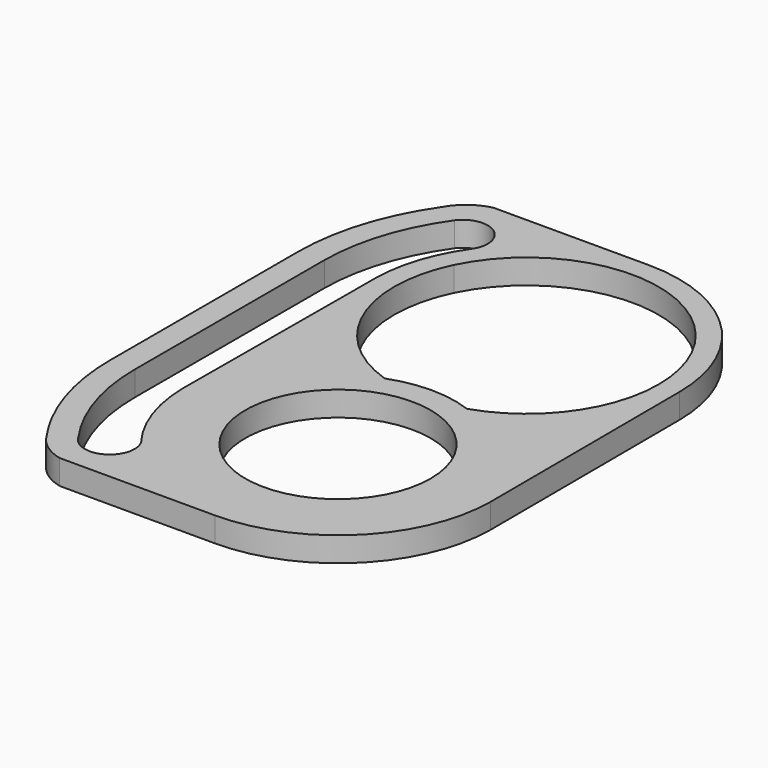
from build123d import *

# Parameters (mm, degrees)
F0_R     = 11.938
F1_DEPTH = 3.175


# Not quite as in the source:
# - a feature names something its author has since deleted; it is built from what else it names


with BuildPart() as f1:
    # F0 (on Top) → F1 (new body)
    with BuildSketch(Plane.XY):
        with BuildLine():
            ThreePointArc((19.6894808556, 0.0781131055), (13.8950303962, 13.9502648114), (0, 19.6896358021))
            Line((0, 19.6896358021), (-20.0037127642, 19.6896358021))
            ThreePointArc((-20.0037127642, 19.6896358021), (-22.390015477, 18.5774210568), (-24.1276545988, 16.5995250638))
            ThreePointArc((-24.1276545988, 16.5995250638), (-28.0183229898, 8.6377085048), (-29.3558392303, -0.1223641979))
            Line((-29.3558392303, -0.1223641979), (-29.3558392303, -30.3483641979))
            ThreePointArc((-29.3558392303, -30.3483641979), (-28.5482645978, -37.1866304526), (-26.1699732087, -43.6486573967))
            ThreePointArc((-26.1699732087, -43.6486573967), (-25.2069369553, -45.3941485327), (-24.1276545988, -47.0702534596))
            ThreePointArc((-24.1276545988, -47.0702534596), (-22.390015477, -49.0481494526), (-20.0037127642, -50.1603641979))
            Line((-20.0037127642, -50.1603641979), (0, -50.1603641979))
            ThreePointArc((0, -50.1603641979), (13.9381398986, -44.4282647716), (19.8109856608, -30.5488415012))
            Line((19.8109856608, -30.5488415012), (19.6894808556, 0.0781131055))
        make_face()
        with BuildLine():
            Line((-19.6805191444, 0.5991028516), (-19.8109856608, -30.5488415012))
            ThreePointArc((-19.8109856608, -30.5488415012), (-18.7320573688, -36.8001368793), (-15.7326179982, -42.3899618877))
            ThreePointArc((-15.7326179982, -42.3899618877), (-15.4201129826, -44.616632299), (-16.6477696645, -46.5003996883))
            ThreePointArc((-16.6477696645, -46.5003996883), (-19.2439967199, -47.0478700205), (-21.3627294259, -45.4506566945))
            ThreePointArc((-21.3627294259, -45.4506566945), (-24.9332630835, -38.2716109559), (-26.1619083245, -30.3483641979))
            Line((-26.1619083245, -30.3483641979), (-26.1434258244, 0.1322556929))
            ThreePointArc((-26.1434258244, 0.1322556929), (-24.8969528592, 7.9773393892), (-21.3520418939, 15.0859707133))
            ThreePointArc((-21.3520418939, 15.0859707133), (-19.3084814881, 16.3545849229), (-16.9550367483, 15.8577761045))
            ThreePointArc((-16.9550367483, 15.8577761045), (-15.5712636207, 13.7334477776), (-16.1488403601, 11.2648441198))
            ThreePointArc((-16.1488403601, 11.2648441198), (-18.6915825929, 6.1892243613), (-19.6805191444, 0.5991028516))
        make_face(mode=Mode.SUBTRACT)
        with Locations((0, -30.3483641979)):
            Circle(F0_R, mode=Mode.SUBTRACT)
        with BuildLine():
            ThreePointArc((-15.3116747346, 7.469335274), (0, 17.0363832022), (15.3116747346, 7.469335274))
            ThreePointArc((15.3116747346, 7.469335274), (15.6883641196, -6.6418057683), (5.2940419625, -16.1929451402))
            ThreePointArc((5.2940419625, -16.1929451402), (0, -15.2353641979), (-5.2940419625, -16.1929451402))
            ThreePointArc((-5.2940419625, -16.1929451402), (-15.6883641196, -6.6418057683), (-15.3116747346, 7.469335274))
        make_face(mode=Mode.SUBTRACT)
    extrude(amount=F1_DEPTH)


solid = f1.part
